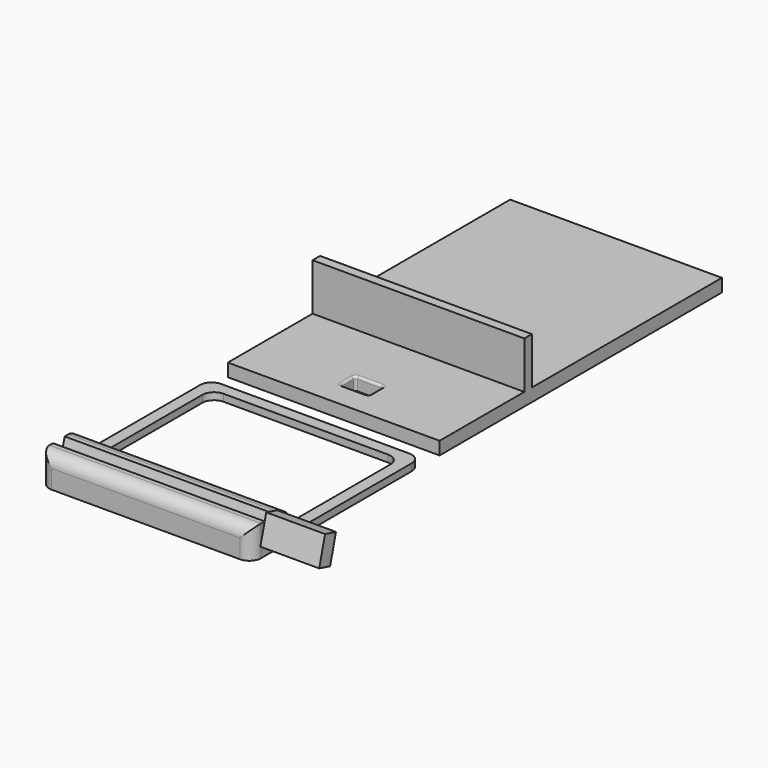
from build123d import *

# Parameters (mm, degrees)
F0_W        = 90
F0_H        = 90
F1_DEPTH    = 3
F2_W        = 20
F2_H        = 10
F3_DEPTH    = 90
F4_W        = 6
F4_H        = 12
F5_DEPTH    = 25
F6_ANGLE    = 15
F8_DEPTH    = 200
F9_T1_DEPTH = 28
F9_T3_DEPTH = 38
F9_T5_DEPTH = 115
F10_W       = 40
F10_H       = 60
F11_DEPTH   = 25
F12_R       = 5
F13_W       = 90
F13_H       = 150
F14_DEPTH   = 5.5
F15_W       = 90
F15_H       = 4
F16_DEPTH   = 20
F17_W       = 12
F17_H       = 8
F18_DEPTH   = 25
F19_R       = 1


# Not quite as in the source:
# - a fillet or chamfer that OpenCascade refuses, or shapes differently, is made with other operations: its cross-section is extruded or revolved along the edge and cut away or added
# - a pattern or mirror of a feature is missing from the dataset's text; its kind, count and spacing are read off the source's solid
# - a feature names something its author has since deleted; it is built from what else it names


with BuildPart() as f1:
    # F0 (on Top) → F1 (new body)
    with BuildSketch(Plane.XY):
        Rectangle(F0_W, F0_H)
    extrude(amount=F1_DEPTH)

    # F2 (on face) → F3 (join, through all)
    with BuildSketch(Plane.YZ.offset(45)):
        with Locations((-35, 8)):
            Rectangle(F2_W, F2_H)
    extrude(amount=-F3_DEPTH)



with BuildPart() as f5:
    # F4 (on face) → F5 (new body)
    with BuildSketch(Plane.YZ.offset(45)):
        with Locations((-35.6848337948, 7)):
            Rectangle(F4_W, F4_H)
    extrude(amount=F5_DEPTH)


with BuildPart() as f5_1:
    # F6: moved
    add(f5.part.rotate(Axis((57.5, -32.6848337948, 13), (-1, 0, 0)), F6_ANGLE))


with BuildPart() as f5_2:
    # F7: moved
    add(f5_1.part.moved(Location((0, 1.2, 1.5))))


with BuildPart() as f1_1:
    add(f1.part)
    # F8 (cut): a face of the model
    f8_faces = [f5_2.part.faces().sort_by_distance(p)[0] for p in [
        (45, -35.9355255443, 9.4809021776),
    ]]
    extrude(f8_faces, amount=F8_DEPTH, mode=Mode.SUBTRACT)

    # F9: fillet of radius 5 on 6 edges, made by hand

    # F9_s2 → F9_t1 (cut)
    with BuildSketch(Plane.XY.offset(-12.5)):
        with BuildLine():
            ThreePointArc((-45, 40), (-43.5355339059, 43.5355339059), (-40, 45))
            Line((-40, 45), (-45, 45))
            Line((-45, 45), (-45, 40))
        make_face()
        with BuildLine():
            ThreePointArc((45, 40), (43.5355339059, 43.5355339059), (40, 45))
            Line((40, 45), (45, 45))
            Line((45, 45), (45, 40))
        make_face()
    extrude(amount=F9_T1_DEPTH, mode=Mode.SUBTRACT)

    # F9_s4 → F9_t3 (cut)
    with BuildSketch(Plane.XY.offset(-12.5)):
        with BuildLine():
            ThreePointArc((-40, -45), (-43.5355339059, -43.5355339059), (-45, -40))
            Line((-45, -40), (-45, -45))
            Line((-45, -45), (-40, -45))
        make_face()
        with BuildLine():
            ThreePointArc((40, -45), (43.5355339059, -43.5355339059), (45, -40))
            Line((45, -40), (45, -45))
            Line((45, -45), (40, -45))
        make_face()
    extrude(amount=F9_T3_DEPTH, mode=Mode.SUBTRACT)

    # F9_s6 → F9_t5 (cut)
    with BuildSketch(Plane.YZ.offset(-57.5)):
        with BuildLine():
            ThreePointArc((-45, 8), (-43.5355339059, 11.5355339059), (-40, 13))
            Line((-40, 13), (-45, 13))
            Line((-45, 13), (-45, 8))
        make_face()
        with BuildLine():
            ThreePointArc((-30, 13), (-26.4644660941, 11.5355339059), (-25, 8))
            Line((-25, 8), (-25, 13))
            Line((-25, 13), (-30, 13))
        make_face()
    extrude(amount=F9_T5_DEPTH, mode=Mode.SUBTRACT)

    # F10 (on face) → F11 (cut)
    with BuildSketch(Plane.XY.offset(3)):
        with Locations((-20, 10)):
            Rectangle(F10_W, F10_H)
    f11 = extrude(amount=-F11_DEPTH, mode=Mode.SUBTRACT)

    # F11_copies: F11 across plane
    add(f11.mirror(Plane(origin=(0, 0, 0), x_dir=(0, 0, 1), z_dir=(1, 0, 0))), mode=Mode.SUBTRACT)

    # F12
    f12_edges = [f1_1.edges().sort_by_distance(p)[0] for p in [
        (-40, 40, 1.5),
        (-40, -20, 1.5),
        (40, 40, 1.5),
        (40, -20, 1.5),
    ]]
    fillet(f12_edges, radius=F12_R)


with BuildPart() as f14:
    # F13 (on Top) → F14 (new body)
    with BuildSketch(Plane.XY):
        with Locations((0.1279246807, 129.6591617167)):
            Rectangle(F13_W, F13_H)
    extrude(amount=F14_DEPTH)

    # F15 (on face) → F16 (join)
    with BuildSketch(Plane.XY.offset(5.5)):
        with Locations((0.1279246807, 101.6591617167)):
            Rectangle(F15_W, F15_H)
    extrude(amount=F16_DEPTH)

    # F17 (on face) → F18 (cut)
    with BuildSketch(Plane.XY.offset(5.5)):
        with Locations((0.1279246807, 69.6591617167)):
            Rectangle(F17_W, F17_H)
    extrude(amount=-F18_DEPTH, mode=Mode.SUBTRACT)

    # F19
    f19_edges = [f14.edges().sort_by_distance(p)[0] for p in [
        (-5.872075, 73.659162, 2.75),
        (6.127925, 73.659162, 2.75),
        (0.127925, 65.659162, 5.5),
        (-5.872075, 69.659162, 5.5),
        (6.127925, 65.659162, 2.75),
        (-5.872075, 65.659162, 2.75),
        (6.127925, 69.659162, 5.5),
        (0.127925, 73.659162, 5.5),
    ]]
    fillet(f19_edges, radius=F19_R)


solid = Compound([f5_2.part, f1_1.part, f14.part])
